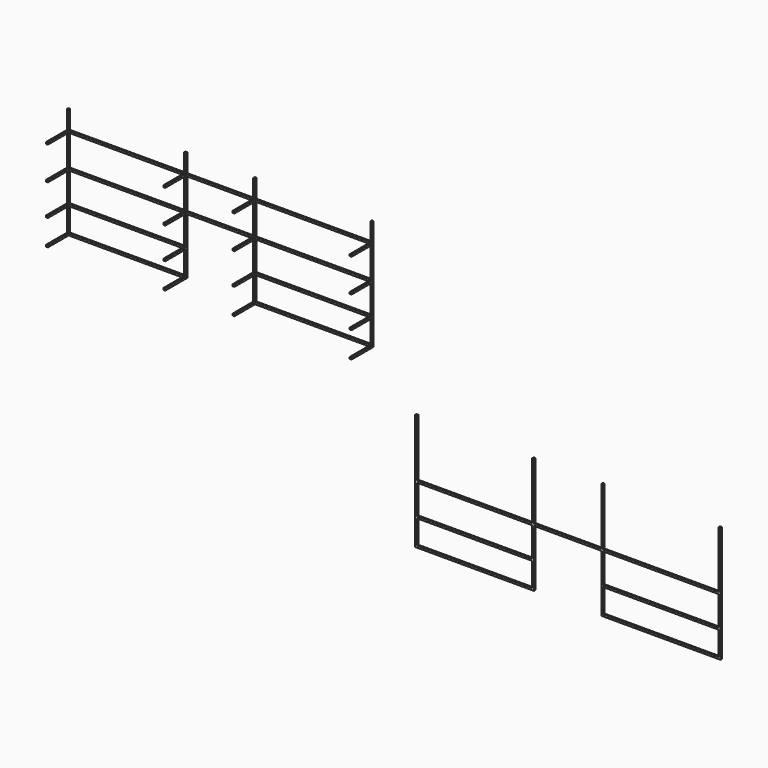
from build123d import *

# Parameters (mm, degrees)
F0_W     = 20
F0_H     = 20
F0_W_2   = 1250
F0_H_2   = 260
F0_H_3   = 320
F0_H_4   = 340
F0_W_3   = 730
F0_H_5   = 200
F1_DEPTH = 20
F0_H_6   = 620
F0_H_7   = 280
F2_W     = 20
F2_H     = 20
F3_DEPTH = 280


with BuildPart() as f1:
    # F0 (on Front) → F1 (new body)
    with BuildSketch(Plane.XZ):
        with Locations((10, 10)):
            Rectangle(F0_W, F0_H)
        with Locations((645, 10)):
            Rectangle(F0_W_2, F0_H)
        with Locations((10, 150)):
            Rectangle(F0_W, F0_H_2)
        with Locations((1280, 10)):
            Rectangle(F0_W, F0_H)
        with Locations((10, 290)):
            Rectangle(F0_W, F0_H)
        with Locations((1280, 150)):
            Rectangle(F0_W, F0_H_2)
        with Locations((645, 290)):
            Rectangle(F0_W_2, F0_H)
        with Locations((10, 460)):
            Rectangle(F0_W, F0_H_3)
        with Locations((1280, 290)):
            Rectangle(F0_W, F0_H)
        with Locations((10, 630)):
            Rectangle(F0_W, F0_H)
        with Locations((1280, 460)):
            Rectangle(F0_W, F0_H_3)
        with Locations((645, 630)):
            Rectangle(F0_W_2, F0_H)
        with Locations((10, 810)):
            Rectangle(F0_W, F0_H_4)
        with Locations((1280, 630)):
            Rectangle(F0_W, F0_H)
        with Locations((10, 990)):
            Rectangle(F0_W, F0_H)
        with Locations((1655, 630)):
            Rectangle(F0_W_3, F0_H)
        with Locations((1280, 810)):
            Rectangle(F0_W, F0_H_4)
        with Locations((645, 990)):
            Rectangle(F0_W_2, F0_H)
        with Locations((10, 1100)):
            Rectangle(F0_W, F0_H_5)
        with Locations((2030, 460)):
            Rectangle(F0_W, F0_H_3)
        with Locations((2030, 630)):
            Rectangle(F0_W, F0_H)
        with Locations((1280, 990)):
            Rectangle(F0_W, F0_H)
        with Locations((1655, 990)):
            Rectangle(F0_W_3, F0_H)
        with Locations((2030, 810)):
            Rectangle(F0_W, F0_H_4)
        with Locations((2030, 290)):
            Rectangle(F0_W, F0_H)
        with Locations((2665, 630)):
            Rectangle(F0_W_2, F0_H)
        with Locations((1280, 1100)):
            Rectangle(F0_W, F0_H_5)
        Polygon((2020, 1000), (2020, 980), (2040, 980), (3290, 980), (3290, 1000), (2040, 1000), align=None)
        with Locations((2030, 150)):
            Rectangle(F0_W, F0_H_2)
        with Locations((2665, 290)):
            Rectangle(F0_W_2, F0_H)
        with Locations((3300, 630)):
            Rectangle(F0_W, F0_H)
        with Locations((3300, 460)):
            Rectangle(F0_W, F0_H_3)
        with Locations((2030, 1100)):
            Rectangle(F0_W, F0_H_5)
        with Locations((3300, 810)):
            Rectangle(F0_W, F0_H_4)
        with Locations((2030, 10)):
            Rectangle(F0_W, F0_H)
        with Locations((3300, 290)):
            Rectangle(F0_W, F0_H)
        with Locations((3300, 990)):
            Rectangle(F0_W, F0_H)
        with Locations((2665, 10)):
            Rectangle(F0_W_2, F0_H)
        with Locations((3300, 150)):
            Rectangle(F0_W, F0_H_2)
        with Locations((3300, 1100)):
            Rectangle(F0_W, F0_H_5)
        with Locations((3300, 10)):
            Rectangle(F0_W, F0_H)
    extrude(amount=F1_DEPTH)

    # F2 (on face) → F3 (join)
    with BuildSketch(Plane.XZ.offset(20)):
        with Locations((10, 990)):
            Rectangle(F2_W, F2_H)
        with Locations((10, 630)):
            Rectangle(F2_W, F2_H)
        with Locations((10, 290)):
            Rectangle(F2_W, F2_H)
        with Locations((10, 10)):
            Rectangle(F2_W, F2_H)
        with Locations((1280, 290)):
            Rectangle(F2_W, F2_H)
        with Locations((1280, 990)):
            Rectangle(F2_W, F2_H)
        with Locations((1280, 630)):
            Rectangle(F2_W, F2_H)
        with Locations((1280, 10)):
            Rectangle(F2_W, F2_H)
        with Locations((2030, 630)):
            Rectangle(F2_W, F2_H)
        with Locations((2030, 290)):
            Rectangle(F2_W, F2_H)
        with Locations((2030, 10)):
            Rectangle(F2_W, F2_H)
        with Locations((3300, 10)):
            Rectangle(F2_W, F2_H)
        with Locations((3300, 630)):
            Rectangle(F2_W, F2_H)
        with Locations((3300, 290)):
            Rectangle(F2_W, F2_H)
        with Locations((2030, 990)):
            Rectangle(F2_W, F2_H)
        with Locations((3300, 990)):
            Rectangle(F2_W, F2_H)
    extrude(amount=F3_DEPTH)


with BuildPart() as f1b:
    # F0 (on Front) → F1, piece 2 (new body)
    with BuildSketch(Plane.XZ):
        with Locations((3782.2742335002, -1740.5566911344)):
            Rectangle(F0_W, F0_H)
        with Locations((4417.2742335002, -1740.5566911344)):
            Rectangle(F0_W_2, F0_H)
        with Locations((3782.2742335002, -1600.5566911344)):
            Rectangle(F0_W, F0_H_2)
        with Locations((5052.2742335002, -1740.5566911344)):
            Rectangle(F0_W, F0_H)
        with Locations((3782.2742335002, -1460.5566911344)):
            Rectangle(F0_W, F0_H)
        with Locations((5052.2742335002, -1600.5566911344)):
            Rectangle(F0_W, F0_H_2)
        with Locations((4417.2742335002, -1460.5566911344)):
            Rectangle(F0_W_2, F0_H)
        with Locations((3782.2742335002, -1290.5566911344)):
            Rectangle(F0_W, F0_H_3)
        with Locations((5052.2742335002, -1460.5566911344)):
            Rectangle(F0_W, F0_H)
        with Locations((3782.2742335002, -1120.5566911344)):
            Rectangle(F0_W, F0_H)
        with Locations((5052.2742335002, -1290.5566911344)):
            Rectangle(F0_W, F0_H_3)
        with Locations((4417.2742335002, -1120.5566911344)):
            Rectangle(F0_W_2, F0_H)
        with Locations((3782.2742335002, -800.5566911344)):
            Rectangle(F0_W, F0_H_6)
        with Locations((5052.2742335002, -1120.5566911344)):
            Rectangle(F0_W, F0_H)
        with Locations((5427.2742335002, -1120.5566911344)):
            Rectangle(F0_W_3, F0_H)
        with Locations((5052.2742335002, -940.5566911344)):
            Rectangle(F0_W, F0_H_4)
        with Locations((5802.2742335002, -1290.5566911344)):
            Rectangle(F0_W, F0_H_3)
        with Locations((5802.2742335002, -1120.5566911344)):
            Rectangle(F0_W, F0_H)
        with Locations((5052.2742335002, -630.5566911344)):
            Rectangle(F0_W, F0_H_7)
        with Locations((5802.2742335002, -940.5566911344)):
            Rectangle(F0_W, F0_H_4)
        with Locations((5802.2742335002, -1460.5566911344)):
            Rectangle(F0_W, F0_H)
        with Locations((6437.2742335002, -1120.5566911344)):
            Rectangle(F0_W_2, F0_H)
        with Locations((5802.2742335002, -630.5566911344)):
            Rectangle(F0_W, F0_H_7)
        with Locations((5802.2742335002, -1600.5566911344)):
            Rectangle(F0_W, F0_H_2)
        with Locations((6437.2742335002, -1460.5566911344)):
            Rectangle(F0_W_2, F0_H)
        with Locations((7072.2742335002, -1120.5566911344)):
            Rectangle(F0_W, F0_H)
        with Locations((7072.2742335002, -1290.5566911344)):
            Rectangle(F0_W, F0_H_3)
        with Locations((7072.2742335002, -940.5566911344)):
            Rectangle(F0_W, F0_H_4)
        with Locations((5802.2742335002, -1740.5566911344)):
            Rectangle(F0_W, F0_H)
        with Locations((7072.2742335002, -1460.5566911344)):
            Rectangle(F0_W, F0_H)
        with Locations((7072.2742335002, -630.5566911344)):
            Rectangle(F0_W, F0_H_7)
        with Locations((6437.2742335002, -1740.5566911344)):
            Rectangle(F0_W_2, F0_H)
        with Locations((7072.2742335002, -1600.5566911344)):
            Rectangle(F0_W, F0_H_2)
        with Locations((7072.2742335002, -1740.5566911344)):
            Rectangle(F0_W, F0_H)
    extrude(amount=F1_DEPTH)


solid = Compound([f1.part, f1b.part])
